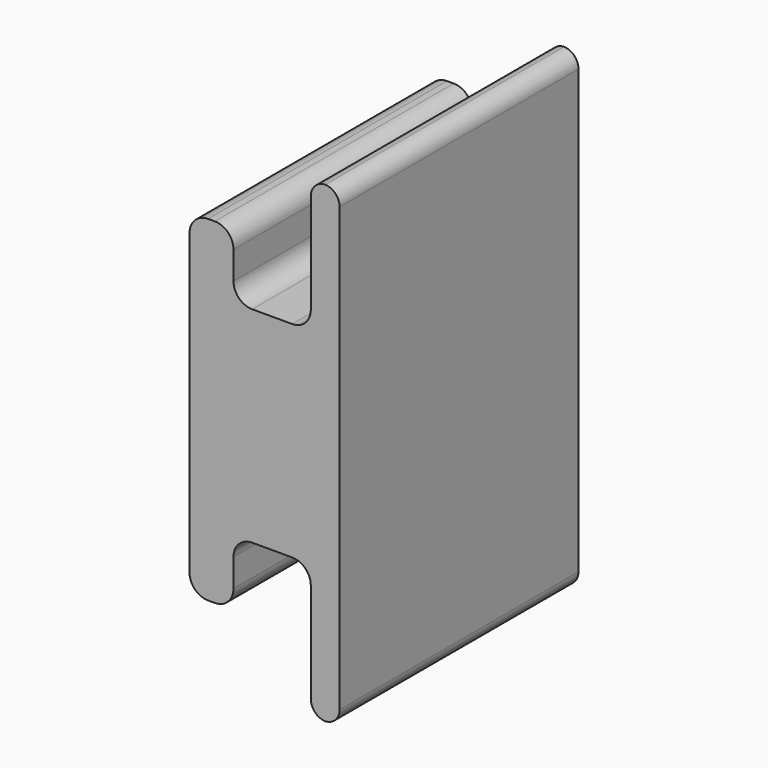
from build123d import *

# Parameters (mm, degrees)
F1_DEPTH    = 40
F2_R        = 2.5
F3_T1_DEPTH = 50


# Not quite as in the source:
# - a fillet or chamfer that OpenCascade refuses, or shapes differently, is made with other operations: its cross-section is extruded or revolved along the edge and cut away or added


with BuildPart() as f1:
    # F0 (on Front) → F1 (new body)
    with BuildSketch(Plane.XZ):
        Polygon((-23.9221176861, 22.5), (-23.9221176861, 0), (-23.9221176861, -22.5), (-18.0304694658, -22.5), (-18.0304694658, -13.7641071746), (-7.6692953279, -13.7641071746), (-7.6692953279, -31.6422108453), (-3.809250768, -31.6422108453), (-3.809250768, 0), (-3.809250768, 31.6422108453), (-7.6692953279, 31.6422108453), (-7.6692953279, 13.7641071746), (-18.0304694658, 13.7641071746), (-18.0304694658, 22.5), align=None)
    extrude(amount=F1_DEPTH)

    # F2
    f2_edges = [f1.edges().sort_by_distance(p)[0] for p in [
        (-23.922118, -20, 22.5),
        (-18.030469, -20, 22.5),
        (-23.922118, -20, -22.5),
        (-18.030469, -20, -22.5),
        (-18.030469, -20, 13.764107),
        (-18.030469, -20, -13.764107),
        (-7.669295, -20, 13.764107),
        (-7.669295, -20, -13.764107),
    ]]
    fillet(f2_edges, radius=F2_R)

    # F3: fillet of radius 2 on 4 edges, made by hand

    # F3_s2 → F3_t1 (cut)
    with BuildSketch(Plane.XZ.offset(-5)):
        with BuildLine():
            ThreePointArc((-7.6692953279, 29.6422108453), (-7.0835088902, 31.0564244077), (-5.6692953279, 31.6422108453))
            Line((-5.6692953279, 31.6422108453), (-7.6692953279, 31.6422108453))
            Line((-7.6692953279, 31.6422108453), (-7.6692953279, 29.6422108453))
        make_face()
        with BuildLine():
            ThreePointArc((-5.809250768, 31.6422108453), (-4.3950372056, 31.0564244077), (-3.809250768, 29.6422108453))
            Line((-3.809250768, 29.6422108453), (-3.809250768, 31.6422108453))
            Line((-3.809250768, 31.6422108453), (-5.809250768, 31.6422108453))
        make_face()
        with BuildLine():
            ThreePointArc((-5.6692953279, -31.6422108453), (-7.0835088902, -31.0564244077), (-7.6692953279, -29.6422108453))
            Line((-7.6692953279, -29.6422108453), (-7.6692953279, -31.6422108453))
            Line((-7.6692953279, -31.6422108453), (-5.6692953279, -31.6422108453))
        make_face()
        with BuildLine():
            ThreePointArc((-3.809250768, -29.6422108453), (-4.3950372056, -31.0564244077), (-5.809250768, -31.6422108453))
            Line((-5.809250768, -31.6422108453), (-3.809250768, -31.6422108453))
            Line((-3.809250768, -31.6422108453), (-3.809250768, -29.6422108453))
        make_face()
    extrude(amount=F3_T1_DEPTH, mode=Mode.SUBTRACT)


solid = f1.part
